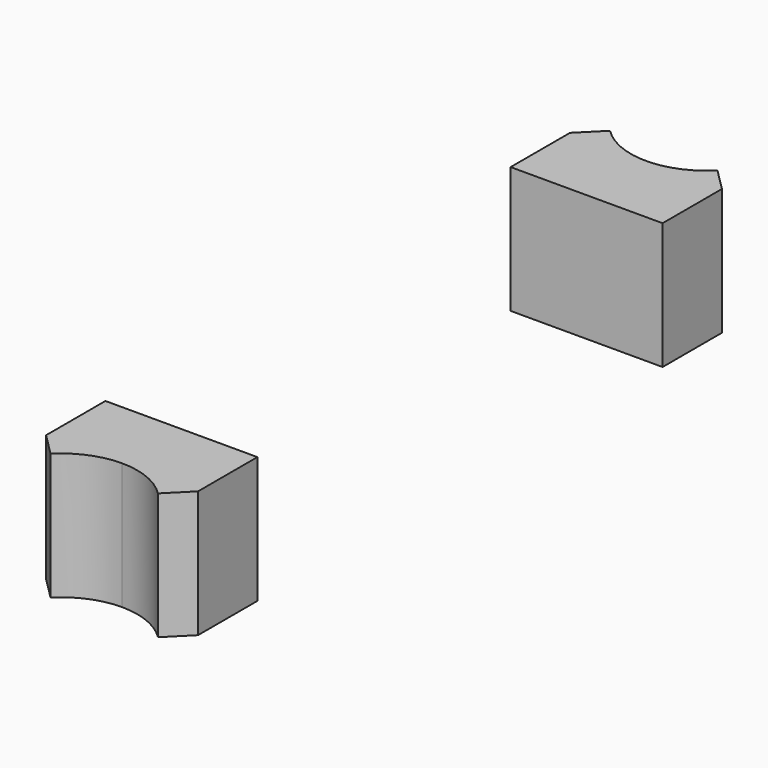
from build123d import *

# Parameters (mm, degrees)
F1_DEPTH = 7


# Not quite as in the source:
# - a feature names something its author has since deleted; it is built from what else it names


with BuildPart() as f1:
    # F0 (on Top) → F1 (new body)
    with BuildSketch(Plane.XY):
        with BuildLine():
            Line((4.2, -18.1), (4.2, -14))
            Line((4.2, -14), (0, -14))
            Line((0, -14), (0, -18.1))
            ThreePointArc((0, -18.1), (1.6072704159, -18.4197059635), (2.969848481, -19.330151519))
            Line((2.969848481, -19.330151519), (4.2, -18.1))
        make_face()
        with BuildLine():
            Line((0, -14), (-4.2, -14))
            Line((-4.2, -14), (-4.2, -18.1))
            Line((-4.2, -18.1), (-2.969848481, -19.330151519))
            ThreePointArc((-2.969848481, -19.330151519), (-1.6072704159, -18.4197059635), (0, -18.1))
            Line((0, -18.1), (0, -14))
        make_face()
    extrude(amount=F1_DEPTH)


with BuildPart() as f1b:
    # F0 (on Top) → F1, piece 2 (new body)
    with BuildSketch(Plane.XY):
        with BuildLine():
            Line((4.2, 14), (4.2, 18.1))
            Line((4.2, 18.1), (2.969848481, 19.330151519))
            ThreePointArc((2.969848481, 19.330151519), (0, 18.1), (-2.969848481, 19.330151519))
            Line((-2.969848481, 19.330151519), (-4.2, 18.1))
            Line((-4.2, 18.1), (-4.2, 14))
            Line((-4.2, 14), (4.2, 14))
        make_face()
    extrude(amount=F1_DEPTH)


solid = Compound([f1.part, f1b.part])
